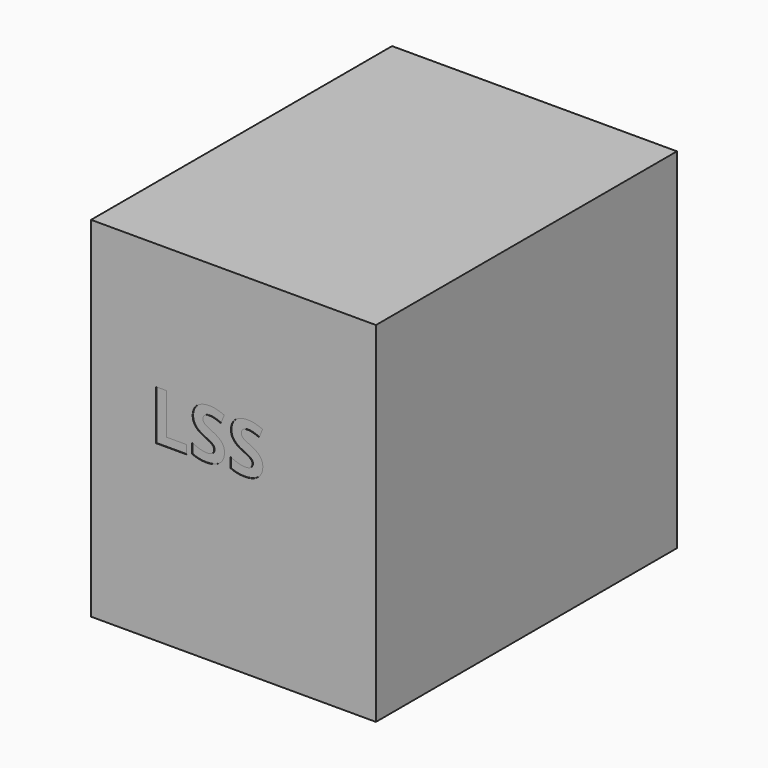
from build123d import *

# Parameters (mm, degrees)
F0_W         = 530
F0_H         = 700
F1_DEPTH     = 650
F2_TEXT_SIZE = 129.4296234846
F3_DEPTH     = 1


# Not quite as in the source:
# - Text() gives the source's letters only with a copy of the font that has no kerning and outlines rounded to 1/6400 em; it was checked with that copy


with BuildPart() as f1:
    # F0 (on Top) → F1 (new body)
    with BuildSketch(Plane.XY):
        with Locations((-9.1542492169, 97.5885838736)):
            Rectangle(F0_W, F0_H)
    extrude(amount=F1_DEPTH)

    # F2 (on face) → F3 (cut)
    with BuildSketch(Plane.XZ.offset(252.4114161264)):
        with Locations((-165.2476638556, 323.4801292419)):
            Text('LSS', F2_TEXT_SIZE, font='Open Sans', font_style=FontStyle.BOLD, text_align=(TextAlign.LEFT, TextAlign.BOTTOM))
    extrude(amount=-F3_DEPTH, mode=Mode.SUBTRACT)


solid = f1.part
